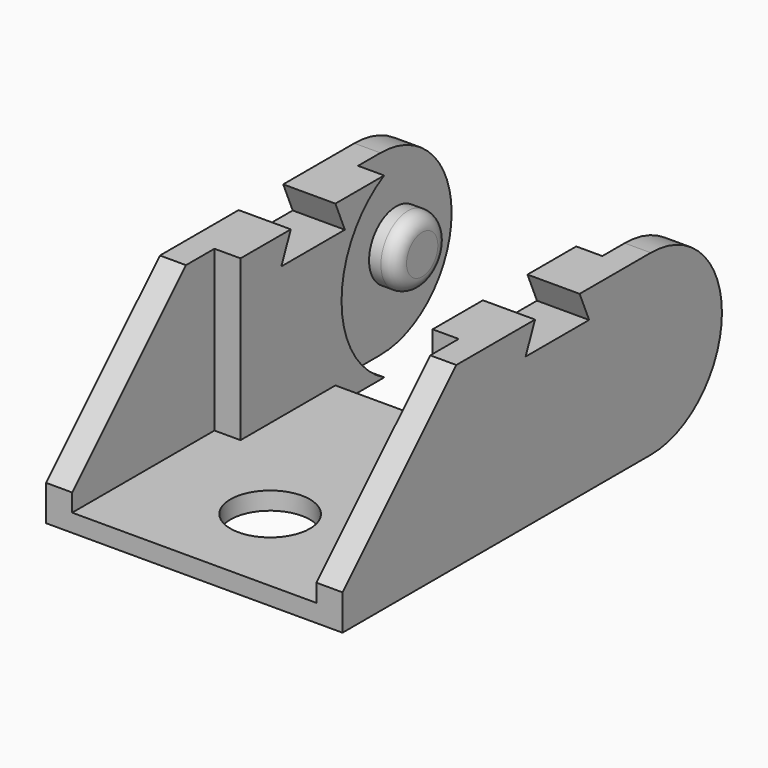
from build123d import *

# Parameters (mm, degrees)
F0_W      = 2.2
F0_H      = 15
F1_DEPTH  = 1.5
F0_W_2    = 4.4
F0_H_2    = 4.6
F2_DEPTH  = 15
F3_SIZE   = 12
F5_DEPTH  = 25
F6_R      = 2.85
F7_DEPTH  = 2.2
F8_R      = 1.2
F9_R      = 7.49999
F10_R     = 3.35
F11_DEPTH = 25


# Not quite as in the source:
# - a fillet or chamfer is up to 0.001 mm smaller than in the source, because OpenCascade refuses the exact size
# - a pattern or mirror of a feature is missing from the dataset's text; its kind, count and spacing are read off the source's solid


with BuildPart() as f1:
    # F0 (on Top) → F1 (new body)
    with BuildSketch(Plane.XY):
        Polygon((8.1, 0.4), (8.1, 5), (-8.1, 5), (-8.1, 0.4), (-8.1, -5), (-8.1, -20), (8.1, -20), (8.1, -5), align=None)
        with Locations((-9.2, -12.5)):
            Rectangle(F0_W, F0_H)
        with Locations((9.2, -12.5)):
            Rectangle(F0_W, F0_H)
    extrude(amount=F1_DEPTH)

    # F0 (on Top) → F2 (join)
    with BuildSketch(Plane.XY):
        with Locations((-10.3, 12.5)):
            Rectangle(F0_W_2, F0_H)
        with Locations((10.3, 12.5)):
            Rectangle(F0_W_2, F0_H)
        with Locations((-10.3, 2.7)):
            Rectangle(F0_W_2, F0_H_2)
        with Locations((10.3, 2.7)):
            Rectangle(F0_W_2, F0_H_2)
        with Locations((-11.4, -12.5)):
            Rectangle(F0_W, F0_H)
        Polygon((-8.1, -5), (-8.1, 0.4), (-12.5, 0.4), (-12.5, -5), (-10.3, -5), align=None)
        Polygon((12.5, -5), (12.5, 0.4), (8.1, 0.4), (8.1, -5), (10.3, -5), align=None)
        with Locations((11.4, -12.5)):
            Rectangle(F0_W, F0_H)
    extrude(amount=F2_DEPTH)

    # F3
    f3_edges = [f1.edges().sort_by_distance(p)[0] for p in [
        (11.4, -20, 15),
        (-11.4, -20, 15),
    ]]
    chamfer(f3_edges, length=F3_SIZE)

    # F4 (on face) → F5 (cut)
    with BuildSketch(Plane.YZ.offset(12.5)):
        Polygon((6, 12.653529644), (5, 15), (0.3, 15), (-0.7, 12.653529644), align=None)
    extrude(amount=-F5_DEPTH, mode=Mode.SUBTRACT)

    # F6 (on face) → F7 (cut)
    with BuildSketch(Plane.YZ.offset(-8.1)):
        with BuildLine():
            Line((20, 1.3383538289), (20, 13.6716461711))
            ThreePointArc((20, 13.6716461711), (19.1242226672, 14.3975416295), (18.1593630584, 15))
            Line((18.1593630584, 15), (10.1406412151, 15))
            ThreePointArc((10.1406412151, 15), (5.6500087774, 7.4943749708), (10.1593912813, 0))
            Line((10.1593912813, 0), (18.1406129922, 0))
            ThreePointArc((18.1406129922, 0), (19.1156030804, 0.6062459626), (20, 1.3383538289))
        make_face()
        with Locations((14.1500021368, 7.505)):
            Circle(F6_R, mode=Mode.SUBTRACT)
    f7 = extrude(amount=-F7_DEPTH, mode=Mode.SUBTRACT)

    # F7_copies: F7 across plane
    add(f7.mirror(Plane(origin=(0, 0, 0), x_dir=(0, 0, 1), z_dir=(1, 0, 0))), mode=Mode.SUBTRACT)

    # F8
    f8_edges = [f1.edges().sort_by_distance(p)[0] for p in [
        (-8.1, 11.300002, 7.505),
        (8.1, 11.300002, 7.505),
    ]]
    fillet(f8_edges, radius=F8_R)

    # F9 (radius 7.5 in the source; OpenCascade refuses exactly that, so slightly less here)
    f9_edges = [f1.edges().sort_by_distance(p)[0] for p in [
        (-10.3, 20, 15),
        (-10.3, 20, 0),
        (10.3, 20, 15),
        (10.3, 20, 0),
    ]]
    fillet(f9_edges, radius=F9_R)

    # F10 (on face) → F11 (cut)
    with BuildSketch(Plane.XY.offset(1.5)):
        with Locations((0, -12)):
            Circle(F10_R)
    extrude(amount=-F11_DEPTH, mode=Mode.SUBTRACT)


solid = f1.part
